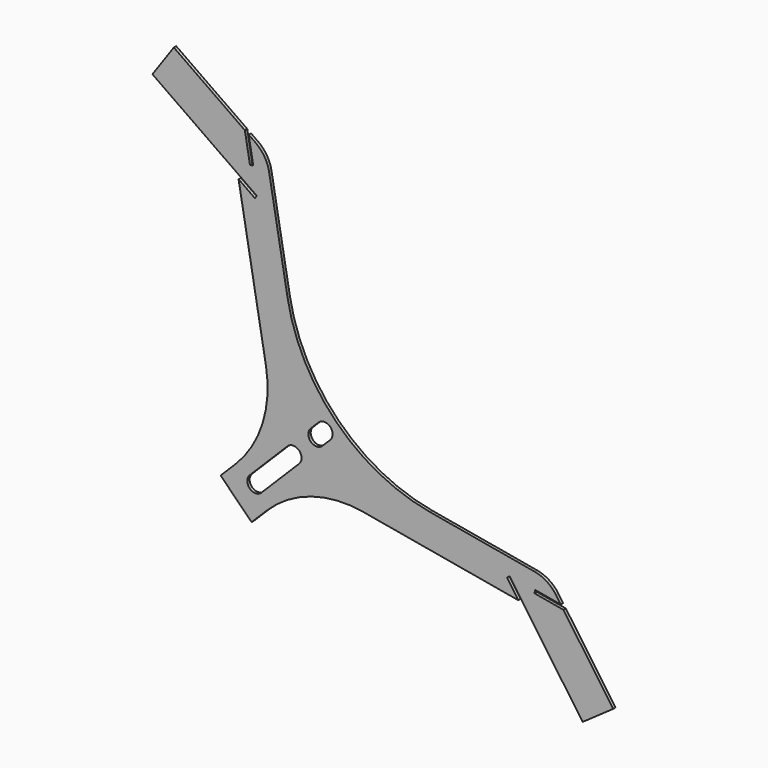
from build123d import *

# Parameters (mm, degrees)
F1_DEPTH = 3.429


# Not quite as in the source:
# - ends of sketch curves that miss each other by under 0.0002 mm in the source are joined


with BuildPart() as f1:
    # F0 (on Front) → F1 (new body)
    with BuildSketch(Plane.XZ):
        with BuildLine():
            Line((-198.875523, -331.3710416), (-198.2139038, -327.6189282))
            Line((-198.2139038, -327.6189282), (-168.4471104, -332.867635))
            Line((-168.4471104, -332.867635), (-174.023655, -324.9035158))
            ThreePointArc((-174.023655, -324.9035158), (-184.7622274276, -314.6235496681), (-198.6173544615, -309.2355853348))
            Line((-198.6173544615, -309.2355853348), (-319.9769826, -287.83661))
            ThreePointArc((-319.9769826, -287.83661), (-428.3757561371, -231.4077731371), (-484.8045910801, -123.0089992615))
            Line((-484.8045910801, -123.0089992615), (-506.203585, -1.649349))
            ThreePointArc((-506.203585, -1.649349), (-511.5915580136, 12.2057554868), (-521.8715008941, 22.9443250094))
            Line((-521.8715008941, 22.9443250094), (-529.835618, 28.5208726))
            Line((-529.835618, 28.5208726), (-524.5869112, -1.2459208))
            Line((-524.5869112, -1.2459208), (-528.33905, -1.9075146))
            Line((-528.33905, -1.9075146), (-534.2493252, 31.6113922))
            Line((-534.2493252, 31.6113922), (-616.5409056, 89.2325622))
            Line((-616.5409056, 89.2325622), (-641.3079376, 53.861589))
            Line((-641.3079376, 53.861589), (-520.4086366, -30.7930042))
            Line((-520.4086366, -30.7930042), (-522.5939764, -33.9139784))
            Line((-522.5939764, -33.9139784), (-541.541589, -20.6467202))
            Line((-541.541589, -20.6467202), (-509.8508218, -200.3739452))
            ThreePointArc((-509.8508218, -200.3739452), (-513.7993593908, -260.6169022992), (-545.1188511893, -312.2298278107))
            Line((-545.1188511893, -312.2298278107), (-562.3549332, -329.4659146))
            Line((-562.3549332, -329.4659146), (-526.4338976, -365.3869248))
            Line((-526.4338976, -365.3869248), (-509.1978386, -348.1508658))
            ThreePointArc((-509.1978386, -348.1508658), (-457.5849106992, -316.8313763908), (-397.341954706, -312.8828450725))
            Line((-397.341954706, -312.8828450725), (-217.6147032, -344.573606))
            Line((-217.6147032, -344.573606), (-230.8819614, -325.6259934))
            Line((-230.8819614, -325.6259934), (-227.7609872, -323.4406536))
            Line((-227.7609872, -323.4406536), (-143.106394, -444.3399292))
            Line((-143.106394, -444.3399292), (-107.7354208, -419.5728972))
            Line((-107.7354208, -419.5728972), (-165.3565908, -337.2813422))
            Line((-165.3565908, -337.2813422), (-198.875523, -331.3710416))
        make_face()
        with BuildLine():
            ThreePointArc((-484.9002250908, -274.4618325092), (-471.4298472592, -274.4618261592), (-471.4298282092, -287.9322039908))
            Line((-471.4298282092, -287.9322039908), (-515.2085708, -331.7109698))
            ThreePointArc((-515.2085708, -331.7109698), (-528.6789538908, -331.7109708908), (-528.6789538908, -318.2405867092))
            Line((-528.6789538908, -318.2405867092), (-484.9002250908, -274.4618325092))
        make_face(mode=Mode.SUBTRACT)
        with BuildLine():
            ThreePointArc((-448.9791894908, -238.5408223092), (-435.5088053092, -238.5408223092), (-435.5088053092, -252.0112064908))
            Line((-435.5088053092, -252.0112064908), (-444.4890526, -260.9914516))
            ThreePointArc((-444.4890526, -260.9914516), (-457.9594356908, -260.9914526908), (-457.9594356908, -247.5210685092))
            Line((-457.9594356908, -247.5210685092), (-448.9791894908, -238.5408223092))
        make_face(mode=Mode.SUBTRACT)
    extrude(amount=F1_DEPTH)


solid = f1.part
